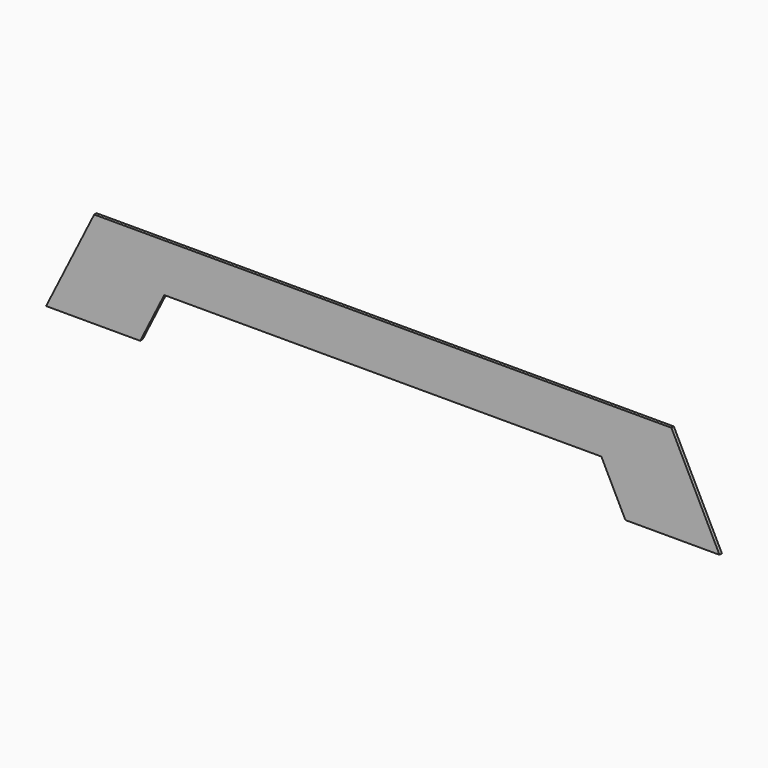
from build123d import *

# Parameters (mm, degrees)
F1_DEPTH = 3.175


# Not quite as in the source:
# - ends of sketch curves that miss each other by under 0.0002 mm in the source are joined


with BuildPart() as f1:
    # F0 (on Front) → F1 (new body)
    with BuildSketch(Plane.XZ):
        Polygon((0, -50.8), (0, 0), (-304.8, -6.031e-07), (-355.6, -101.6), (-256.2067782821, -101.6), (-230.8067781314, -50.8), align=None)
        Polygon((304.8, 0), (0, -3.015e-07), (0, -50.8), (230.8067784001, -50.8), (256.2067784001, -101.6), (355.6, -101.6), align=None)
    extrude(amount=F1_DEPTH)


solid = f1.part
